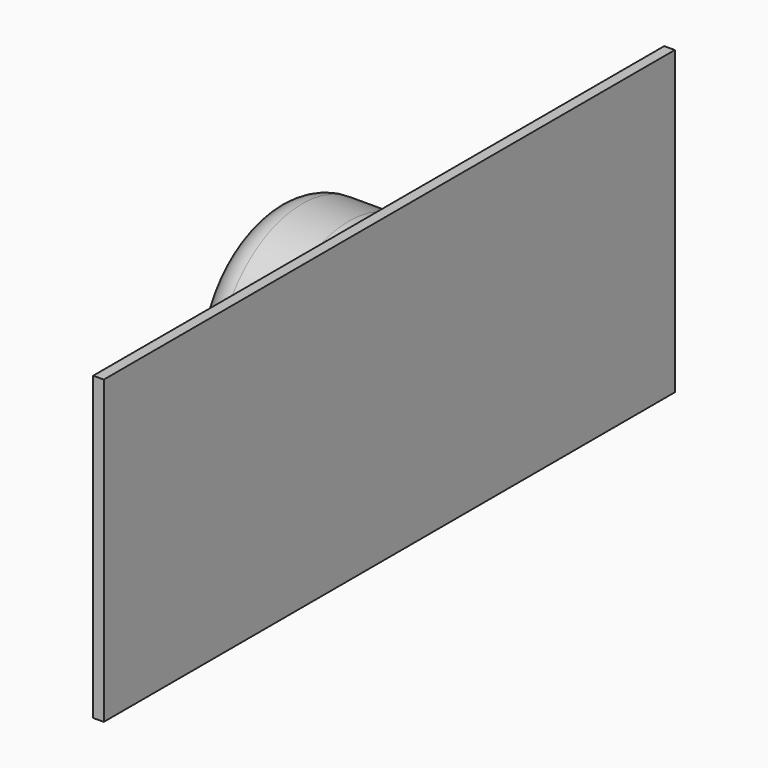
from build123d import *

# Parameters (mm, degrees)
F0_W          = 11.3538
F0_H          = 6.4262
F2_R          = 3.175
F3_DEPTH      = 38.1
F5_DEPTH      = 11.3538
F6_W          = 5.3086
F6_H          = 1.8508250259
F7_DEPTH      = 1.5748
F8_W          = 1.5748
F8_H          = 12.7
F9_DEPTH      = 2.54
F10_SIZE      = 1.27
F11_TEXT_SIZE = 1.7638888889
F12_DEPTH     = 0.508


# Not quite as in the source:
# - Text() gives the source's letters only with a copy of the font that has no kerning and outlines rounded to 1/6400 em; it was checked with that copy


with BuildPart() as f1:
    # F0 (on Front) → F1 (revolve)
    with BuildSketch(Plane.XZ):
        with Locations((-5.6769, 8.1661)):
            Rectangle(F0_W, F0_H)
    revolve(axis=Axis((-6.9125968808, 0, 0), (1, 0, 0)))

    # F2
    f2_edges = [f1.edges().sort_by_distance(p)[0] for p in [
        (-11.3538, 0, -4.953),
        (-11.3538, 0, -11.3792),
        (0, 0, -11.3792),
        (-5.6769, 0, 11.3792),
    ]]
    fillet(f2_edges, radius=F2_R)


with BuildPart() as f3:
    # F0 (on Front) → F3 (new body, symmetric)
    with BuildSketch(Plane.XZ):
        Polygon((0, 13.36543262), (0, 11.3792), (0, 4.953), (0, -18.8072640449), (1.1300308397, -18.8072640449), (1.1300308397, 13.36543262), align=None)
    extrude(amount=F3_DEPTH, both=True)


with BuildPart() as f5:
    # F4 (on Right) → F5 (new body)
    with BuildSketch(Plane.YZ):
        Polygon((0.7874, -11.4412640449), (0, -11.4412640449), (-0.7874, -11.4412640449), (-0.7874, -17.7912640449), (0.7874, -17.7912640449), align=None)
    extrude(amount=-F5_DEPTH)

    # F6 (on face) → F7 (cut, through all)
    with BuildSketch(Plane(origin=(0, 0.7874, 0), x_dir=(-1, 0, 0), z_dir=(0, 1, 0))):
        with Locations((2.6543, -12.3666765578)):
            Rectangle(F6_W, F6_H)
    extrude(amount=-F7_DEPTH, mode=Mode.SUBTRACT)

    # F8 (on face) → F9 (join)
    with BuildSketch(Plane(origin=(-11.3538, 0, 0), x_dir=(0, -1, 0), z_dir=(-1, 0, 0))):
        with Locations((0, -11.4412640449)):
            Rectangle(F8_W, F8_H)
    extrude(amount=F9_DEPTH)

    # F10
    f10_edges = [f5.edges().sort_by_distance(p)[0] for p in [
        (-11.3538, 0, -11.441264),
    ]]
    chamfer(f10_edges, length=F10_SIZE)

    # F11 (on face) → F12 (cut)
    with BuildSketch(Plane(origin=(0, 0.7874, 0), x_dir=(-1, 0, 0), z_dir=(0, 1, 0))):
        with Locations((6.4182441566, -16.6984443883)):
            Text('B09892', F11_TEXT_SIZE, font='Open Sans', font_style=FontStyle.BOLD, text_align=(TextAlign.LEFT, TextAlign.BOTTOM))
    extrude(amount=-F12_DEPTH, mode=Mode.SUBTRACT)


solid = Compound([f1.part, f3.part, f5.part])
